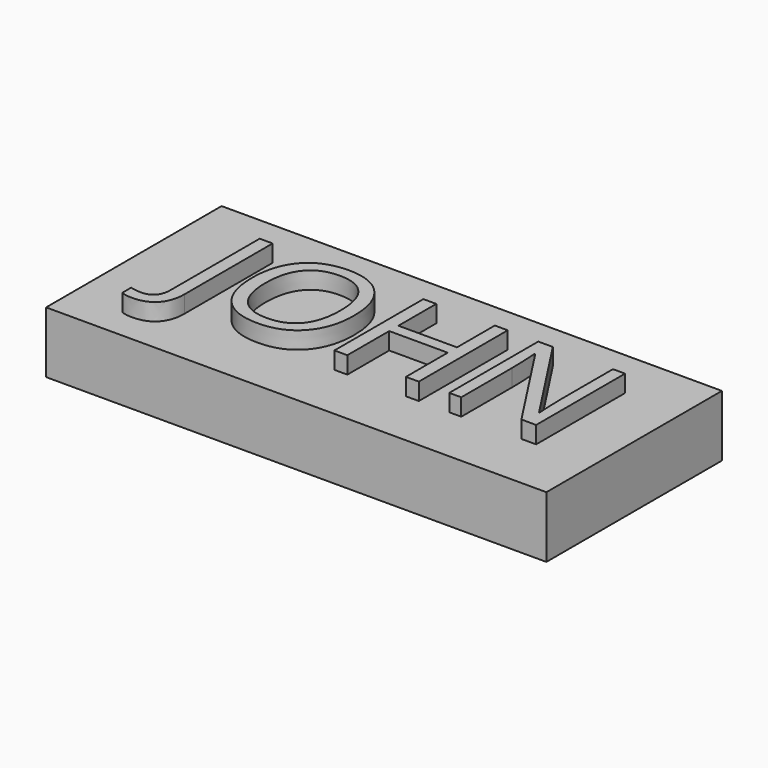
from build123d import *

# Parameters (mm, degrees)
F0_TEXT_SIZE = 64.4062024852
F1_DEPTH     = 7.0781819522
F2_W         = 206.9554142654
F2_H         = 90.7590761781
F3_DEPTH     = 25.4


# Not quite as in the source:
# - Text() gives the source's letters only with a copy of the font that has no kerning and outlines rounded to 1/6400 em; it was checked with that copy


with BuildPart() as f1:
    # F0 (on Top) → F1 (new body)
    with BuildSketch(Plane.XY):
        with Locations((0, 0)):
            Text('JOHN', F0_TEXT_SIZE, font='Open Sans', text_align=(TextAlign.LEFT, TextAlign.BOTTOM))
    extrude(amount=F1_DEPTH)

    # F2 (on Top) → F3 (join)
    with BuildSketch(Plane.XY):
        with Locations((77.1123841405, 21.3369615376)):
            Rectangle(F2_W, F2_H)
    extrude(amount=-F3_DEPTH)


solid = f1.part
